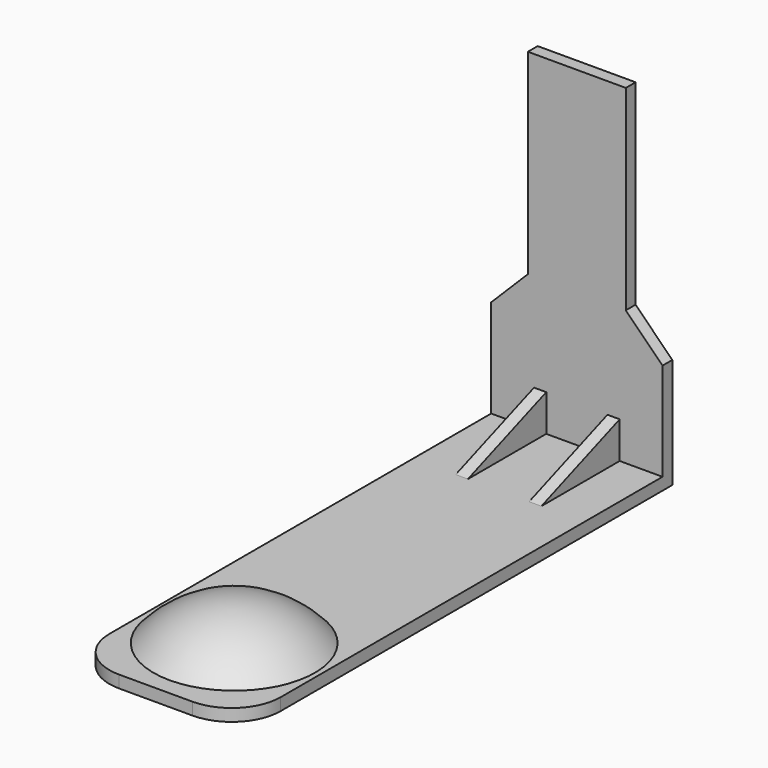
from build123d import *

# Parameters (mm, degrees)
F0_W     = 139.7
F0_H     = 3.175
F1_DEPTH = 22.225
F4_R     = 12.7
F6_DEPTH = 3.175
F9_DEPTH = 1.5875


# Not quite as in the source:
# - a pattern or mirror of a feature is missing from the dataset's text; its kind, count and spacing are read off the source's solid


with BuildPart() as f1:
    # F0 (on Right) → F1 (new body, symmetric)
    with BuildSketch(Plane.YZ):
        with Locations((44.45, -1.5875)):
            Rectangle(F0_W, F0_H)
    extrude(amount=F1_DEPTH, both=True)

    # F2 (on Right) → F3 (revolve)
    with BuildSketch(Plane.YZ):
        with BuildLine():
            Line((0, 0), (0, 9.525))
            ThreePointArc((0, 9.525), (-11.5091012898, 7.0320228377), (-20.955, 0))
            Line((-20.955, 0), (0, 0))
        make_face()
    revolve(axis=Axis((0, 0, 4.7625), (0, 0, -1)))

    # F4
    f4_edges = [f1.edges().sort_by_distance(p)[0] for p in [
        (22.225, -25.4, -1.5875),
        (-22.225, -25.4, -1.5875),
    ]]
    fillet(f4_edges, radius=F4_R)

    # F5 (on face) → F6 (join)
    with BuildSketch(Plane(origin=(0, 114.3, 0), x_dir=(-1, 0, 0), z_dir=(0, 1, 0))):
        Polygon((-22.225, 25.4), (-22.225, 0), (22.225, 0), (22.225, 25.4), (12.7, 34.925), (12.7, 85.725), (-12.7, 85.725), (-12.7, 34.925), align=None)
    extrude(amount=-F6_DEPTH)

    # F8 (on offset) → F9 (join, symmetric)
    with BuildSketch(Plane.YZ.offset(9.525)):
        Polygon((111.125, 0), (111.125, 9.525), (85.725, 0), align=None)
    f9 = extrude(amount=F9_DEPTH, both=True)

    # F9_copies: F9 across plane
    add(f9.mirror(Plane(origin=(0, 0, 0), x_dir=(0, 0, -1), z_dir=(-1, 0, 0))))


solid = f1.part
